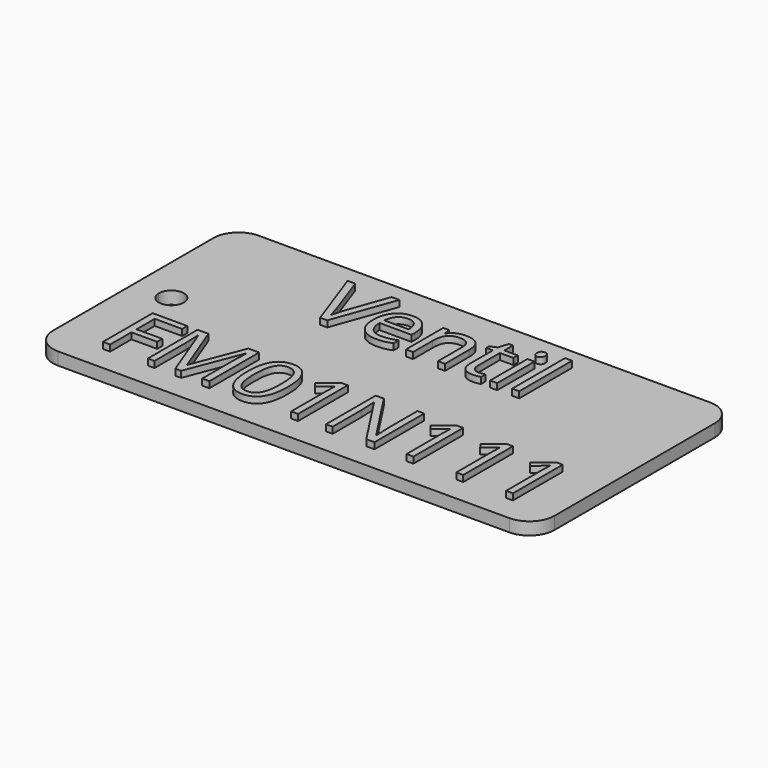
from build123d import *

# Parameters (mm, degrees)
F1_DEPTH     = 2
F2_TEXT_SIZE = 13.8888888889
F3_DEPTH     = 1


# Not quite as in the source:
# - Text() gives the source's letters only with a copy of the font that has no kerning and outlines rounded to 1/6400 em; it was checked with that copy


with BuildPart() as f1:
    # F0 (on Top) → F1 (new body)
    with BuildSketch(Plane.XY):
        with BuildLine():
            Line((-36, -20), (36, -20))
            ThreePointArc((36, -20), (38.8284271247, -18.8284271247), (40, -16))
            Line((40, -16), (40, 16))
            ThreePointArc((40, 16), (38.8284271247, 18.8284271247), (36, 20))
            Line((36, 20), (-36, 20))
            ThreePointArc((-36, 20), (-38.8284271247, 18.8284271247), (-40, 16))
            Line((-40, 16), (-40, 0))
            Line((-40, 0), (-40, -16))
            ThreePointArc((-40, -16), (-38.8284271247, -18.8284271247), (-36, -20))
        make_face()
        with BuildLine():
            ThreePointArc((-32, 0), (-34, -1.9063982912), (-36, 0))
            ThreePointArc((-36, 0), (-34.0479635482, 2.0976228847), (-31.9977021381, 0.0958995707))
            ThreePointArc((-31.9977021381, 0.0958995707), (-31.998276686, 0.0479360225), (-32, 0))
        make_face(mode=Mode.SUBTRACT)
    extrude(amount=F1_DEPTH)

    # F2 (on face) → F3 (join)
    with BuildSketch(Plane.XY.offset(2)):
        with Locations((-18.5423865914, 6)):
            Text('Ventil', F2_TEXT_SIZE, font='Open Sans', text_align=(TextAlign.LEFT, TextAlign.BOTTOM))
        with Locations((-33.4095116705, -16)):
            Text('FM01N111', F2_TEXT_SIZE, font='Open Sans', text_align=(TextAlign.LEFT, TextAlign.BOTTOM))
    extrude(amount=F3_DEPTH)


solid = f1.part
